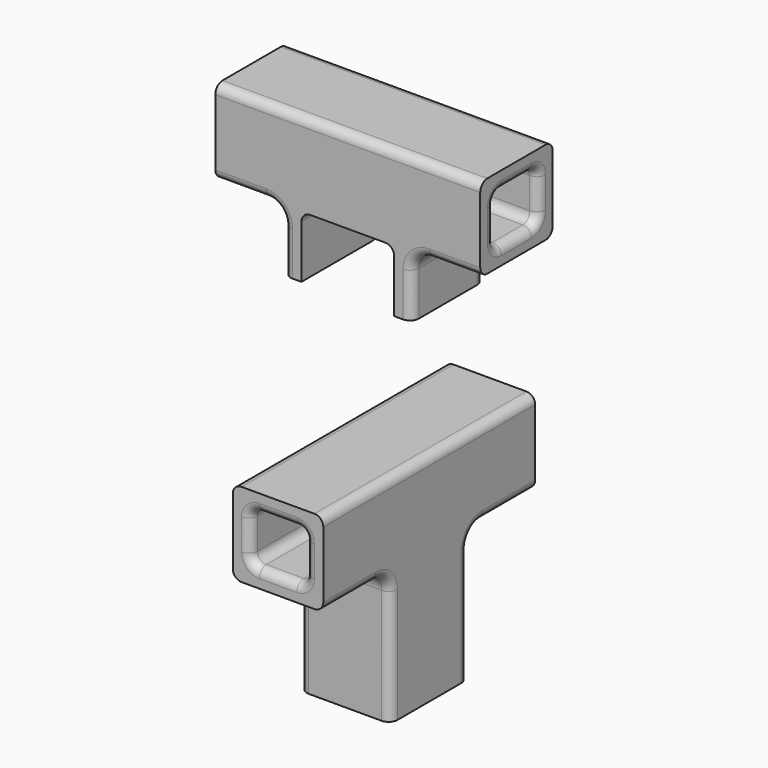
from build123d import *

# Parameters (mm, degrees)
F0_W       = 10.25
F0_H       = 9.5
F0_W_2     = 6.25
F0_H_2     = 5.5
F1_DEPTH   = 15
F2_W       = 10.25
F2_H       = 9.5
F2_W_2     = 6.25
F2_H_2     = 5.5
F3_DEPTH   = 15
F4_W       = 2
F4_H       = 10.25
F5_DEPTH   = 7
F6_W       = 10.25
F6_H       = 11
F6_W_2     = 5.25
F6_H_2     = 6
F7_DEPTH   = 15
F8_R       = 2
F9_R       = 2
F10_F1_R   = 1
F10_F2_R   = 1
F10_2_F1_R = 1
F10_2_F2_R = 1
F11_R      = 1
F11_2_R    = 1
F12_R      = 1
F12_2_R    = 1
F13_R      = 1


with BuildPart() as f1:
    # F0 (on Front) → F1 (new body, symmetric)
    with BuildSketch(Plane.XZ):
        Rectangle(F0_W, F0_H)
        Rectangle(F0_W_2, F0_H_2, mode=Mode.SUBTRACT)
    extrude(amount=F1_DEPTH, both=True)

    # F6 (on face) → F7 (join)
    with BuildSketch(Plane(origin=(0, 0, -4.75), x_dir=(1, 0, 0), z_dir=(0, 0, -1))):
        Rectangle(F6_W, F6_H)
        Rectangle(F6_W_2, F6_H_2, mode=Mode.SUBTRACT)
    extrude(amount=F7_DEPTH)

    # F9
    f9_edges = [f1.edges().sort_by_distance(p)[0] for p in [
        (0, -5.5, -4.75),
        (0, 5.5, -4.75),
    ]]
    fillet(f9_edges, radius=F9_R)

    # F10#2: fillet of radius 1 on 6 edges, made by hand

    # F10_2_f1
    f10_2_f1_edges = [f1.edges().sort_by_distance(p)[0] for p in [
        (3.125, 0, 2.75),
        (-3.125, 0, 2.75),
        (-3.125, 0, -2.75),
        (3.125, 0, -2.75),
    ]]
    fillet(f10_2_f1_edges, radius=F10_2_F1_R)

    # F10_2_f2
    f10_2_f2_edges = [f1.edges().sort_by_distance(p)[0] for p in [
        (0, -15, 2.75),
        (0, 15, 2.75),
        (-2.8321067812, 15, 2.4571067812),
        (2.8321067812, 15, 2.4571067812),
        (-2.8321067812, -15, 2.4571067812),
        (2.8321067812, -15, 2.4571067812),
    ]]
    fillet(f10_2_f2_edges, radius=F10_2_F2_R)

    # F11#2
    f11_2_edges = [f1.edges().sort_by_distance(p)[0] for p in [
        (-5.125, 0, 4.75),
        (5.125, 0, 4.75),
    ]]
    fillet(f11_2_edges, radius=F11_2_R)

    # F12#2
    f12_2_edges = [f1.edges().sort_by_distance(p)[0] for p in [
        (-5.125, -11.25, -4.75),
        (-5.125, 11.25, -4.75),
        (5.125, -11.25, -4.75),
        (5.125, 11.25, -4.75),
    ]]
    fillet(f12_2_edges, radius=F12_2_R)

    # F13
    f13_edges = [f1.edges().sort_by_distance(p)[0] for p in [
        (-2.625, -3, -12.25),
        (2.625, -3, -12.25),
        (2.625, 3, -12.25),
        (-2.625, 3, -12.25),
    ]]
    fillet(f13_edges, radius=F13_R)


with BuildPart() as f3:
    # F2 (on Right) → F3 (new body, symmetric)
    with BuildSketch(Plane.YZ):
        with Locations((0, 7.5550233014)):
            Rectangle(F2_W, F2_H)
        with Locations((0, 7.5550233014)):
            Rectangle(F2_W_2, F2_H_2, mode=Mode.SUBTRACT)
    extrude(amount=F3_DEPTH, both=True)

    # F4 (on face) → F5 (join)
    with BuildSketch(Plane(origin=(0, 0, 2.8050233014), x_dir=(1, 0, 0), z_dir=(0, 0, -1))):
        with Locations((-6.25, 0)):
            Rectangle(F4_W, F4_H)
        with Locations((6.25, 0)):
            Rectangle(F4_W, F4_H)
    extrude(amount=F5_DEPTH)

    # F8
    f8_edges = [f3.edges().sort_by_distance(p)[0] for p in [
        (7.25, 0, 2.805023),
        (-7.25, 0, 2.805023),
    ]]
    fillet(f8_edges, radius=F8_R)

    # F10: fillet of radius 1 on 6 edges, made by hand

    # F10_f1
    f10_f1_edges = [f3.edges().sort_by_distance(p)[0] for p in [
        (0, -3.125, 10.3050233014),
        (0, 3.125, 4.8050233014),
        (0, -3.125, 4.8050233014),
        (0, 3.125, 10.3050233014),
    ]]
    fillet(f10_f1_edges, radius=F10_F1_R)

    # F10_f2
    f10_f2_edges = [f3.edges().sort_by_distance(p)[0] for p in [
        (15, 0, 10.3050233014),
        (-15, 0, 10.3050233014),
        (-15, -2.8321067812, 10.0121300826),
        (-15, 2.8321067812, 10.0121300826),
        (15, -2.8321067812, 10.0121300826),
        (15, 2.8321067812, 10.0121300826),
    ]]
    fillet(f10_f2_edges, radius=F10_F2_R)

    # F11
    f11_edges = [f3.edges().sort_by_distance(p)[0] for p in [
        (0, 5.125, 12.305023),
        (0, -5.125, 12.305023),
        (-5.25, 0, 2.805023),
        (5.25, 0, 2.805023),
    ]]
    fillet(f11_edges, radius=F11_R)

    # F12
    f12_edges = [f3.edges().sort_by_distance(p)[0] for p in [
        (-12.125, 5.125, 2.805023),
        (12.125, 5.125, 2.805023),
        (-12.125, -5.125, 2.805023),
        (12.125, -5.125, 2.805023),
    ]]
    fillet(f12_edges, radius=F12_R)


with BuildPart() as f3_1:
    # F14: moved
    add(f3.part.moved(Location((0, 0, 25))))


solid = Compound([f1.part, f3_1.part])
